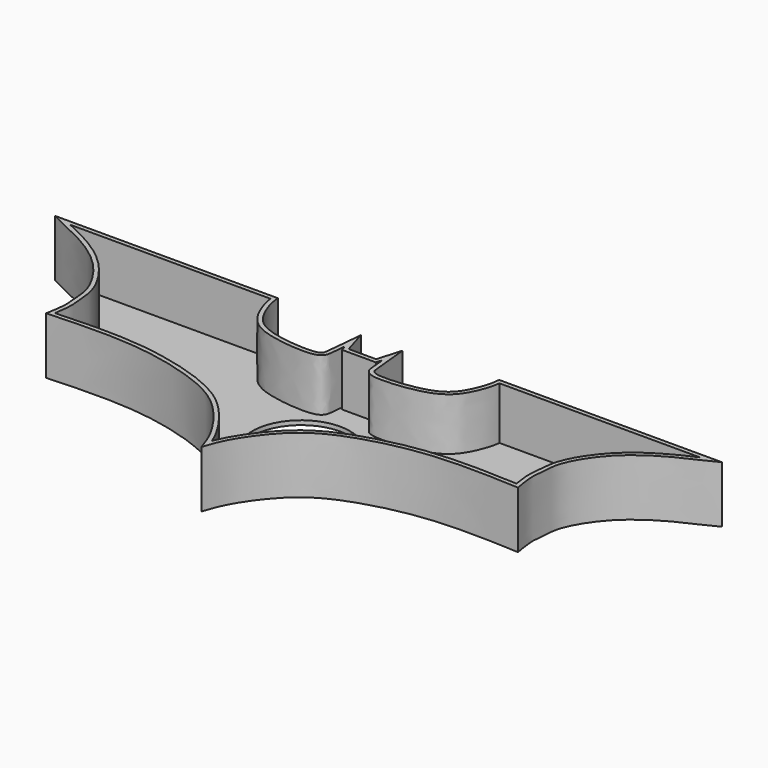
from build123d import *

# Parameters (mm, degrees)
F1_DEPTH = 10
F2_T     = -0.762
F3_R     = 8.5831388835
F4_DEPTH = 25.4


with BuildPart() as f1:
    # F0 (on Top) → F1 (new body)
    with BuildSketch(Plane.XY):
        with BuildLine():
            Line((-19.4826032966, 17.2526277602), (-58.6904734373, 17.2526277602))
            add(Edge.make_bspline(
                [(-58.6904734373, 17.2526277602), (-58.281111495, 17.0224612469), (-57.1314465146, 16.3760543568), (-52.0348771848, 14.2545396551), (-45.3232929877, 9.8859671938), (-41.3070106136, 3.2601674122), (-41.3014742082, 0.0389783097), (-40.8669091385, -2.337023355), (-41.2861365471, -4.7810910017), (-41.5234342217, -6.1645205133)],
                knots=[0, 0, 0, 0, 0.0883383683, 0.2480922577, 0.4492409467, 0.6381309473, 0.7581185457, 0.8630864646, 1, 1, 1, 1], degree=3))
            add(Edge.make_bspline(
                [(0, -23.8783750683), (-0.4136806457, -22.6242616948), (-1.4001195089, -19.6337757164), (-6.5075660626, -12.5927103472), (-13.036248837, -8.8351170222), (-23.6589286603, -6.0295039138), (-33.7398672705, -5.7706697258), (-39.0559327407, -6.0396642093), (-41.5234342217, -6.1645205133)],
                knots=[0, 0, 0, 0, 0.1228273843, 0.2928870534, 0.4551436553, 0.6490615045, 0.8371086168, 1, 1, 1, 1], degree=3))
            add(Edge.make_bspline(
                [(0, -23.8783750683), (0.4136806457, -22.6242616948), (1.4001195089, -19.6337757164), (6.5075660626, -12.5927103472), (13.036248837, -8.8351170222), (23.6589286603, -6.0295039138), (33.7398672705, -5.7706697258), (39.0559327407, -6.0396642093), (41.5234342217, -6.1645205133)],
                knots=[0, 0, 0, 0, 0.1228273843, 0.2928870534, 0.4551436553, 0.6490615045, 0.8371086168, 1, 1, 1, 1], degree=3))
            add(Edge.make_bspline(
                [(58.6904734373, 17.2526277602), (58.281111495, 17.0224612469), (57.1314465146, 16.3760543568), (52.0348771848, 14.2545396551), (45.3232929877, 9.8859671938), (41.3070106136, 3.2601674122), (41.3014742082, 0.0389783097), (40.8669091385, -2.337023355), (41.2861365471, -4.7810910017), (41.5234342217, -6.1645205133)],
                knots=[0, 0, 0, 0, 0.0883383683, 0.2480922577, 0.4492409467, 0.6381309473, 0.7581185457, 0.8630864646, 1, 1, 1, 1], degree=3))
            Line((58.6904734373, 17.2526277602), (19.4826032966, 17.2526277602))
            add(Edge.make_bspline(
                [(19.4826032966, 17.2526277602), (19.4252067793, 16.7154920348), (19.2857896628, 15.4107802242), (17.9748731189, 11.7943312114), (15.071616289, 8.5153700592), (6.6784902248, 7.6523240998), (4.4257272401, 8.2261943399), (4.2604921057, 9.6627038856), (3.9206068542, 13.2350100378), (3.6801933311, 15.7618355006)],
                knots=[0, 0, 0, 0, 0.1015967646, 0.2467802687, 0.40542182, 0.6239049233, 0.7293914618, 0.8085884816, 1, 1, 1, 1], degree=3))
            Line((3.6801933311, 15.7618355006), (2.4130183738, 11.5130729973))
            Line((2.4130183738, 11.5130729973), (0, 11.5130729973))
            Line((0, 11.5130729973), (-2.4130183738, 11.5130729973))
            Line((-2.4130183738, 11.5130729973), (-3.6801933311, 15.7618355006))
            add(Edge.make_bspline(
                [(-19.4826032966, 17.2526277602), (-19.4252067793, 16.7154920348), (-19.2857896628, 15.4107802242), (-17.9748731189, 11.7943312114), (-15.071616289, 8.5153700592), (-6.6784902248, 7.6523240998), (-4.4257272401, 8.2261943399), (-4.2604921057, 9.6627038856), (-3.9206068542, 13.2350100378), (-3.6801933311, 15.7618355006)],
                knots=[0, 0, 0, 0, 0.1015967646, 0.2467802687, 0.40542182, 0.6239049233, 0.7293914618, 0.8085884816, 1, 1, 1, 1], degree=3))
        make_face()
    extrude(amount=F1_DEPTH)

    # F2
    f2_openings = [f1.faces().sort_by_distance(p)[0] for p in [
        (0, 3.287592, 10),
    ]]
    offset(amount=F2_T, openings=f2_openings, kind=Kind.INTERSECTION)

    # F3 (on face) → F4 (cut)
    with BuildSketch(Plane.XY.offset(0.762)):
        with Locations((0, -1.9574905746)):
            Circle(F3_R)
    extrude(amount=-F4_DEPTH, mode=Mode.SUBTRACT)


solid = f1.part
